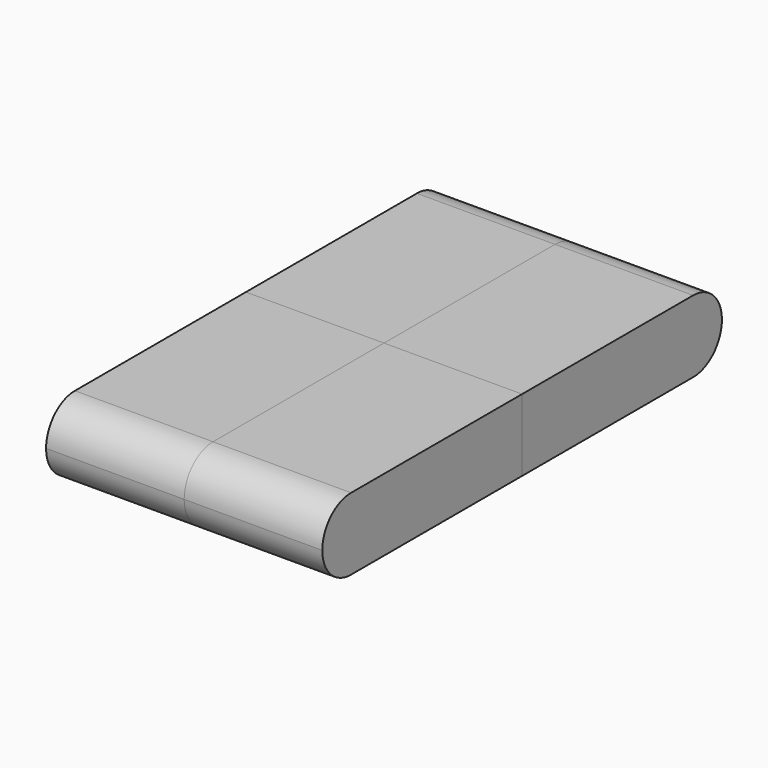
from build123d import *

# Parameters (mm, degrees)
F0_W     = 28.75
F0_H     = 52
F1_DEPTH = 7.5
F2_DEPTH = 7.5
F3_R     = 7.49999
F3_2_R   = 7.49999
F3_3_R   = 7.49999
F3_4_R   = 7.49999


# Not quite as in the source:
# - a fillet or chamfer is up to 0.001 mm smaller than in the source, because OpenCascade refuses the exact size


with BuildPart() as f1:
    # F0 (on Top) → F1 (new body, symmetric)
    with BuildSketch(Plane.XY):
        with Locations((-14.375, 26)):
            Rectangle(F0_W, F0_H)
    extrude(amount=F1_DEPTH, both=True)

    # F3 (radius 7.5 in the source; OpenCascade refuses exactly that, so slightly less here)
    f3_edges = [f1.edges().sort_by_distance(p)[0] for p in [
        (-14.375, 52, 7.5),
        (-14.375, 52, -7.5),
    ]]
    fillet(f3_edges, radius=F3_R)


with BuildPart() as f1b:
    # F0 (on Top) → F1, piece 2 (new body, symmetric)
    with BuildSketch(Plane.XY):
        with Locations((14.375, -26)):
            Rectangle(F0_W, F0_H)
    extrude(amount=F1_DEPTH, both=True)

    # F3#3 (radius 7.5 in the source; OpenCascade refuses exactly that, so slightly less here)
    f3_3_edges = [f1b.edges().sort_by_distance(p)[0] for p in [
        (14.375, -52, 7.5),
        (14.375, -52, -7.5),
    ]]
    fillet(f3_3_edges, radius=F3_3_R)


with BuildPart() as f2:
    # F0 (on Top) → F2 (new body, symmetric)
    with BuildSketch(Plane.XY):
        with Locations((14.375, 26)):
            Rectangle(F0_W, F0_H)
    extrude(amount=F2_DEPTH, both=True)

    # F3#2 (radius 7.5 in the source; OpenCascade refuses exactly that, so slightly less here)
    f3_2_edges = [f2.edges().sort_by_distance(p)[0] for p in [
        (14.375, 52, 7.5),
        (14.375, 52, -7.5),
    ]]
    fillet(f3_2_edges, radius=F3_2_R)


with BuildPart() as f2b:
    # F0 (on Top) → F2, piece 2 (new body, symmetric)
    with BuildSketch(Plane.XY):
        with Locations((-14.375, -26)):
            Rectangle(F0_W, F0_H)
    extrude(amount=F2_DEPTH, both=True)

    # F3#4 (radius 7.5 in the source; OpenCascade refuses exactly that, so slightly less here)
    f3_4_edges = [f2b.edges().sort_by_distance(p)[0] for p in [
        (-14.375, -52, 7.5),
        (-14.375, -52, -7.5),
    ]]
    fillet(f3_4_edges, radius=F3_4_R)


solid = Compound([f1.part, f1b.part, f2.part, f2b.part])
